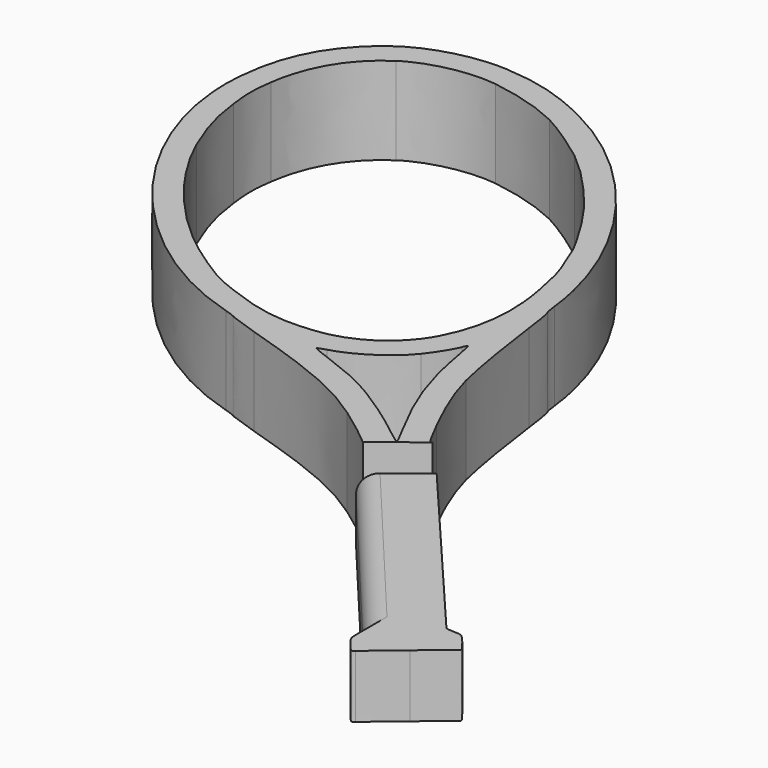
from build123d import *

# Parameters (mm, degrees)
F1_DEPTH = 8.89
F2_DEPTH = 6.35
F3_R     = 1.905


# Not quite as in the source:
# - ends of sketch curves that miss each other by under 0.0002 mm in the source are joined


with BuildPart() as f1:
    # F0 (on Top) → F1 (new body)
    with BuildSketch(Plane.XY):
        with BuildLine():
            add(Edge.make_bspline(
                [(-3.0718564333, -18.3105251546), (-3.1941043079, -18.1127221958), (-5.8648991557, -16.0549205163), (-7.190032708, -15.1375407302)],
                knots=[0, 0, 0, 0, 1, 1, 1, 1], degree=3))
            Line((-3.0718564333, -18.3105251546), (1.283406037, -14.8964376977))
            add(Edge.make_bspline(
                [(-0.3091913774, -12.3824247468), (0.9372726753, -14.8364748026), (1.0557331488, -15.0572735167), (1.283406037, -14.8964376977)],
                knots=[0, 0, 0, 0, 0.9260782938, 0.9260782938, 0.9260782938, 0.9260782938], degree=3))
            add(Edge.make_bspline(
                [(-3.2852139041, -4.9409408201), (-2.7741749014, -6.9668684755), (-1.7162384362, -9.6122164693), (-0.3091913774, -12.3824247468)],
                knots=[0, 0, 0, 0, 1, 1, 1, 1], degree=3))
            add(Edge.make_bspline(
                [(-5.0088641769, 5.214134072), (-4.5421366646, 1.5230281787), (-3.7736378691, -3.0046688221), (-3.2852139041, -4.9409408201)],
                knots=[0, 0, 0, 0, 1, 1, 1, 1], degree=3))
            add(Edge.make_bspline(
                [(-5.4962642413, 8.1725191805), (-5.4284659352, 8.1292535314), (-5.209134736, 6.7979795013), (-5.0088641769, 5.214134072)],
                knots=[0, 0, 0, 0, 1, 1, 1, 1], degree=3))
            add(Edge.make_bspline(
                [(-5.7512520457, 9.4060414253), (-5.6788081565, 8.7708691083), (-5.5640640102, 8.2157848295), (-5.4962642413, 8.1725191805)],
                knots=[0, 0, 0, 0, 1, 1, 1, 1], degree=3))
            add(Edge.make_bspline(
                [(-24.7858665687, 36.1856603825), (-14.96957989, 31.3065842999), (-6.9645844345, 20.044433944), (-5.7512520457, 9.4060414253)],
                knots=[0, 0, 0, 0, 1, 1, 1, 1], degree=3))
            add(Edge.make_bspline(
                [(-34.1873844826, 38.8286343898), (-30.857190368, 38.6418193466), (-28.2565370959, 37.91071925), (-24.7858665687, 36.1856603825)],
                knots=[0, 0, 0, 0, 1, 1, 1, 1], degree=3))
            add(Edge.make_bspline(
                [(-43.9407502785, 36.0908808342), (-41.5350315808, 37.926858848), (-37.633680143, 39.0219614404), (-34.1873844826, 38.8286343898)],
                knots=[0, 0, 0, 0, 1, 1, 1, 1], degree=3))
            add(Edge.make_bspline(
                [(-49.9400395659, 24.5883530034), (-49.5200575018, 29.6066446383), (-47.591125408, 33.3050156546), (-43.9407502785, 36.0908808342)],
                knots=[0, 0, 0, 0, 1, 1, 1, 1], degree=3))
            add(Edge.make_bspline(
                [(-41.4642537241, 3.0200614686), (-47.346464372, 9.6510447366), (-50.5152946856, 17.7147515638), (-49.9400395659, 24.5883530034)],
                knots=[0, 0, 0, 0, 1, 1, 1, 1], degree=3))
            add(Edge.make_bspline(
                [(-25.6339560793, -7.4778913882), (-31.3499205662, -5.8250379875), (-36.8584747989, -2.1720080301), (-41.4642537241, 3.0200614686)],
                knots=[0, 0, 0, 0, 1, 1, 1, 1], degree=3))
            add(Edge.make_bspline(
                [(-24.5267699977, -7.9004054122), (-24.5700619756, -7.8315905191), (-25.0682963705, -7.6414595008), (-25.6339560793, -7.4778913882)],
                knots=[0, 0, 0, 0, 1, 1, 1, 1], degree=3))
            add(Edge.make_bspline(
                [(-21.6470497057, -8.9038118596), (-23.187603157, -8.4207516708), (-24.4834780198, -7.9692203053), (-24.5267699977, -7.9004054122)],
                knots=[0, 0, 0, 0, 1, 1, 1, 1], degree=3))
            add(Edge.make_bspline(
                [(-7.190032708, -15.1375407302), (-10.7579448987, -12.6675020629), (-13.7273003701, -11.3871436816), (-21.6470497057, -8.9038118596)],
                knots=[0, 0, 0, 0, 1, 1, 1, 1], degree=3))
        make_face()
        with BuildLine():
            add(Edge.make_bspline(
                [(-1.8833126768, -14.7865827274), (-4.4917885492, -9.9482767191), (-5.6255492381, -6.7828355163), (-6.456100795, -2.0194497738)],
                knots=[0, 0, 0, 0, 1, 1, 1, 1], degree=3))
            add(Edge.make_bspline(
                [(-0.9901101081, -16.6060803306), (-0.9587568106, -16.5747255704), (-1.3606992098, -15.7559517952), (-1.8833126768, -14.7865827274)],
                knots=[0, 0, 0, 0, 1, 1, 1, 1], degree=3))
            add(Edge.make_bspline(
                [(-2.2673265775, -15.6841339481), (-1.5962109631, -16.222559365), (-1.0214648683, -16.6374336281), (-0.9901101081, -16.6060803306)],
                knots=[0, 0, 0, 0, 1, 1, 1, 1], degree=3))
            add(Edge.make_bspline(
                [(-8.2114715068, -11.5076991948), (-6.4771053834, -12.5491537866), (-4.0445458643, -14.258304165), (-2.2673265775, -15.6841339481)],
                knots=[0, 0, 0, 0, 1, 1, 1, 1], degree=3))
            add(Edge.make_bspline(
                [(-14.2179213331, -8.7620177236), (-11.5463497835, -9.7393073935), (-9.9131035297, -10.4859005681), (-8.2114715068, -11.5076991948)],
                knots=[0, 0, 0, 0, 1, 1, 1, 1], degree=3))
            add(Edge.make_bspline(
                [(-16.0348884392, -8.0120266618), (-16.0348884392, -8.0589549494), (-15.2172541191, -8.3964515854), (-14.2179213331, -8.7620177236)],
                knots=[0, 0, 0, 0, 1, 1, 1, 1], degree=3))
            add(Edge.make_bspline(
                [(-15.1778280971, -7.6916920617), (-15.6492114315, -7.8209478042), (-16.0348884392, -7.9650983743), (-16.0348884392, -8.0120266618)],
                knots=[0, 0, 0, 0, 1, 1, 1, 1], degree=3))
            add(Edge.make_bspline(
                [(-8.9386120338, -3.5958675359), (-10.3003163882, -5.3265329902), (-12.9888530557, -7.091462545), (-15.1778280971, -7.6916920617)],
                knots=[0, 0, 0, 0, 1, 1, 1, 1], degree=3))
            add(Edge.make_bspline(
                [(-7.1114600427, -0.6481543967), (-7.3253938232, -1.2674679568), (-8.1376877706, -2.5779290143), (-8.9386120338, -3.5958675359)],
                knots=[0, 0, 0, 0, 1, 1, 1, 1], degree=3))
            add(Edge.make_bspline(
                [(-6.8652090354, -0.2024826677), (-6.9159740246, -0.2024826677), (-7.0267863928, -0.4030340681), (-7.1114600427, -0.6481543967)],
                knots=[0, 0, 0, 0, 1, 1, 1, 1], degree=3))
            add(Edge.make_bspline(
                [(-6.456100795, -2.0194497738), (-6.6303452649, -1.0201169878), (-6.8144440462, -0.2024826677), (-6.8652090354, -0.2024826677)],
                knots=[0, 0, 0, 0, 1, 1, 1, 1], degree=3))
        make_face(mode=Mode.SUBTRACT)
        with BuildLine():
            add(Edge.make_bspline(
                [(-18.0232667361, -5.7614800923), (-14.4929980663, -5.4074825676), (-11.2612739302, -3.2632256512), (-9.6901564989, -0.2324434605)],
                knots=[0, 0, 0, 0, 1, 1, 1, 1], degree=3))
            add(Edge.make_bspline(
                [(-27.4851991704, -4.2897795647), (-23.6134609476, -5.7847343365), (-21.5130957224, -6.1114229708), (-18.0232667361, -5.7614800923)],
                knots=[0, 0, 0, 0, 1, 1, 1, 1], degree=3))
            add(Edge.make_bspline(
                [(-31.9297042516, -1.9508528252), (-29.8809728683, -3.3074128108), (-29.4719962723, -3.522636706), (-27.4851991704, -4.2897795647)],
                knots=[0, 0, 0, 0, 1, 1, 1, 1], degree=3))
            add(Edge.make_bspline(
                [(-40.2031110306, 5.3774637621), (-37.5453014358, 2.2869940202), (-35.2221632428, 0.2292332967), (-31.9297042516, -1.9508528252)],
                knots=[0, 0, 0, 0, 1, 1, 1, 1], degree=3))
            add(Edge.make_bspline(
                [(-45.2732778554, 13.3047767972), (-44.3211322576, 11.0337946355), (-42.1552373972, 7.6473737537), (-40.2031110306, 5.3774637621)],
                knots=[0, 0, 0, 0, 1, 1, 1, 1], degree=3))
            add(Edge.make_bspline(
                [(-47.3674528705, 20.6733092726), (-47.0329182325, 17.9711391865), (-46.6187782523, 16.513956106), (-45.2732778554, 13.3047767972)],
                knots=[0, 0, 0, 0, 1, 1, 1, 1], degree=3))
            add(Edge.make_bspline(
                [(-47.3584864272, 25.4023071324), (-47.6275279979, 23.5626747078), (-47.629000952, 22.7858910942), (-47.3674528705, 20.6733092726)],
                knots=[0, 0, 0, 0, 1, 1, 1, 1], degree=3))
            add(Edge.make_bspline(
                [(-41.9187646402, 34.4503054637), (-44.9567550908, 32.4183750085), (-46.7746071395, 29.3947030757), (-47.3584864272, 25.4023071324)],
                knots=[0, 0, 0, 0, 1, 1, 1, 1], degree=3))
            add(Edge.make_bspline(
                [(-33.2446456053, 36.2845311449), (-36.0418833946, 36.6833082287), (-39.7536559892, 35.8984197109), (-41.9187646402, 34.4503054637)],
                knots=[0, 0, 0, 0, 1, 1, 1, 1], degree=3))
            add(Edge.make_bspline(
                [(-26.1139094613, 34.1787509485), (-28.0937222815, 35.156160561), (-30.6734397129, 35.9179776741), (-33.2446456053, 36.2845311449)],
                knots=[0, 0, 0, 0, 1, 1, 1, 1], degree=3))
            add(Edge.make_bspline(
                [(-20.7321594606, 30.6290561427), (-22.0508760819, 31.6813728566), (-25.0136946797, 33.6355877975), (-26.1139094613, 34.1787509485)],
                knots=[0, 0, 0, 0, 1, 1, 1, 1], degree=3))
            add(Edge.make_bspline(
                [(-12.9472943951, 21.8068081356), (-14.7289925155, 24.7161899123), (-18.076815272, 28.5101319886), (-20.7321594606, 30.6290561427)],
                knots=[0, 0, 0, 0, 1, 1, 1, 1], degree=3))
            add(Edge.make_bspline(
                [(-10.6868364683, 17.889246158), (-10.6868364683, 18.0243922541), (-11.5979529085, 19.6034326643), (-12.9472943951, 21.8068081356)],
                knots=[0, 0, 0, 0, 1, 1, 1, 1], degree=3))
            add(Edge.make_bspline(
                [(-9.9375908427, 16.0141712331), (-10.3496757082, 16.9763905496), (-10.6868364683, 17.8201723643), (-10.6868364683, 17.889246158)],
                knots=[0, 0, 0, 0, 1, 1, 1, 1], degree=3))
            add(Edge.make_bspline(
                [(-8.4987311938, 10.9735746561), (-9.04247358, 13.736865754), (-9.2027286429, 14.298268962), (-9.9375908427, 16.0141712331)],
                knots=[0, 0, 0, 0, 1, 1, 1, 1], degree=3))
            add(Edge.make_bspline(
                [(-9.6901564989, -0.2324434605), (-8.0162122096, 2.9967033717), (-7.6348692267, 6.5834401567), (-8.4987311938, 10.9735746561)],
                knots=[0, 0, 0, 0, 1, 1, 1, 1], degree=3))
        make_face(mode=Mode.SUBTRACT)
    extrude(amount=F1_DEPTH)


with BuildPart() as f2:
    # F0 (on Top) → F2 (new body)
    with BuildSketch(Plane.XY):
        with BuildLine():
            add(Edge.make_bspline(
                [(14.8392387831, -42.2726795329), (14.1583273659, -41.4412459588), (14.1336104067, -41.3812834173), (14.1336104067, -40.5607880265)],
                knots=[0, 0, 0, 0, 1, 1, 1, 1], degree=3))
            add(Edge.make_bspline(
                [(15.8334286629, -42.8780753592), (15.5469456777, -43.1324473606), (15.5397842247, -43.1280884697), (14.8392387831, -42.2726795329)],
                knots=[0, 0, 0, 0, 1, 1, 1, 1], degree=3))
            add(Edge.make_bspline(
                [(19.1388385333, -40.1091191658), (17.479571127, -41.4911245427), (15.9921361733, -42.7371559268), (15.8334286629, -42.8780753592)],
                knots=[0, 0, 0, 0, 1, 1, 1, 1], degree=3))
            add(Edge.make_bspline(
                [(22.2594402056, -37.5070046413), (22.2023767653, -37.5561621066), (20.7981059397, -38.7271137889), (19.1388385333, -40.1091191658)],
                knots=[0, 0, 0, 0, 1, 1, 1, 1], degree=3))
            add(Edge.make_bspline(
                [(21.5328657494, -36.4312011115), (21.989545872, -36.9737367577), (22.3165036459, -37.457847176), (22.2594402056, -37.5070046413)],
                knots=[0, 0, 0, 0, 1, 1, 1, 1], degree=3))
            add(Edge.make_bspline(
                [(20.0324638267, -35.4447738606), (20.6954262673, -35.4447738606), (20.7113566971, -35.4552469005), (21.5328657494, -36.4312011115)],
                knots=[0, 0, 0, 0, 1, 1, 1, 1], degree=3))
            add(Edge.make_bspline(
                [(19.0343714231, -35.3200627738), (19.214781237, -35.3886538715), (19.6639210633, -35.4447738606), (20.0324638267, -35.4447738606)],
                knots=[0, 0, 0, 0, 1, 1, 1, 1], degree=3))
            Line((19.0343714231, -35.3200627738), (1.8357417879, -15.0657990511))
            Line((1.8357417879, -15.0657990511), (-2.7312379694, -18.6458515533))
            Line((-2.7312379694, -18.6458515533), (-3.1989166405, -19.0124645636))
            Line((-3.1989166405, -19.0124645636), (14.1336104067, -39.7105102942))
            Line((14.1336104067, -39.7105102942), (14.1336104067, -40.5607880265))
        make_face()
    extrude(amount=F2_DEPTH)

    # F3
    f3_edges = [f2.edges().sort_by_distance(p)[0] for p in [
        (5.467347, -29.361487, 6.35),
    ]]
    fillet(f3_edges, radius=F3_R)


solid = Compound([f1.part, f2.part])
